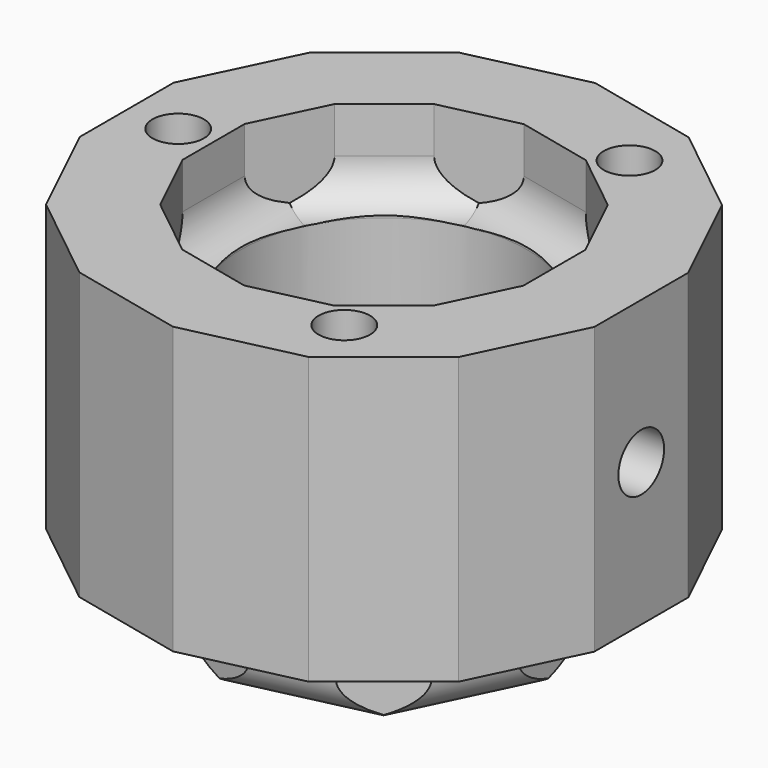
from build123d import *

# Parameters (mm, degrees)
F0_R         = 12.5
F1_DEPTH     = 12.5
F2_R         = 2.25
F3_DEPTH     = 25
F4_R         = 12.5
F5_DEPTH     = 7.5
F6_R         = 12.5
F7_DEPTH     = 7.5
F8_T4_DEPTH  = 24.3016555368
F8_S5_R      = 12.5
F8_T6_DEPTH  = 15
F8_T11_DEPTH = 24.3016555368
F8_S12_R     = 12.5
F8_T13_DEPTH = 14
F8_T17_DEPTH = 24.3016555368
F8_S18_R     = 12.5
F8_T19_DEPTH = 15
F8_T24_DEPTH = 24.3016555368
F8_S25_R     = 12.5
F8_T26_DEPTH = 15
F8_T30_DEPTH = 24.3016555368
F8_S31_R     = 12.5
F8_T32_DEPTH = 15
F8_T37_DEPTH = 24.3016555368
F8_S38_R     = 12.5
F8_T39_DEPTH = 15
F8_T44_DEPTH = 24.3016555368
F8_S45_R     = 12.5
F8_T46_DEPTH = 15
F9_T1_DEPTH  = 24.050587715
F9_T3_DEPTH  = 24.050587715
F9_T5_DEPTH  = 24.050587715
F9_T7_DEPTH  = 24.050587715
F9_T9_DEPTH  = 24.050587715
F9_T11_DEPTH = 24.050587715
F9_T13_DEPTH = 24.050587715
F10_R        = 2.5
F11_DEPTH    = 12


# Not quite as in the source:
# - a fillet or chamfer that OpenCascade refuses, or shapes differently, is made with other operations: its cross-section is extruded or revolved along the edge and cut away or added


with BuildPart() as f1:
    # F0 (on Top) → F1 (new body, symmetric)
    with BuildSketch(Plane.XY):
        Polygon((22.5, -5.1354781738), (22.5, 5.1354781738), (18.0435990556, 14.3892900865), (10.013442028, 20.7931266245), (0, 23.0786294236), (-10.013442028, 20.7931266245), (-18.0435990556, 14.3892900865), (-22.5, 5.1354781738), (-22.5, -5.1354781738), (-18.0435990556, -14.3892900865), (-10.013442028, -20.7931266245), (0, -23.0786294236), (10.013442028, -20.7931266245), (18.0435990556, -14.3892900865), align=None)
        Circle(F0_R, mode=Mode.SUBTRACT)
    extrude(amount=F1_DEPTH, both=True)

    # F2 (on face) → F3 (cut)
    with BuildSketch(Plane.XY.offset(12.5)):
        with Locations((9, 15.5884572681)):
            Circle(F2_R)
        with Locations((-18, 0)):
            Circle(F2_R)
        with Locations((9, -15.5884572681)):
            Circle(F2_R)
    extrude(amount=-F3_DEPTH, mode=Mode.SUBTRACT)

    # F4 (on face) → F5 (cut)
    with BuildSketch(Plane.XY.offset(12.5)):
        Polygon((14.9, -3.4008277684), (14.9, 3.4008277684), (11.9488722635, 9.5289076573), (6.6311238319, 13.7696705203), (0, 15.2831812628), (-6.6311238319, 13.7696705203), (-11.9488722635, 9.5289076573), (-14.9, 3.4008277684), (-14.9, -3.4008277684), (-11.9488722635, -9.5289076573), (-6.6311238319, -13.7696705203), (0, -15.2831812628), (6.6311238319, -13.7696705203), (11.9488722635, -9.5289076573), align=None)
        Circle(F4_R, mode=Mode.SUBTRACT)
    extrude(amount=-F5_DEPTH, mode=Mode.SUBTRACT)

    # F6 (on face) → F7 (join)
    with BuildSketch(Plane(origin=(0, 0, -12.5), x_dir=(1, 0, 0), z_dir=(0, 0, -1))):
        Polygon((14.35, -3.2752938575), (14.35, 3.2752938575), (11.5078065088, 9.1771694552), (6.3863508045, 13.2613940917), (0, 14.719036988), (-6.3863508045, 13.2613940917), (-11.5078065088, 9.1771694552), (-14.35, 3.2752938575), (-14.35, -3.2752938575), (-11.5078065088, -9.1771694552), (-6.3863508045, -13.2613940917), (0, -14.719036988), (6.3863508045, -13.2613940917), (11.5078065088, -9.1771694552), align=None)
        Circle(F6_R, mode=Mode.SUBTRACT)
    extrude(amount=F7_DEPTH)

    # F8: fillet of radius 3.5 on 7 edges, made by hand


with BuildPart() as f8_tool2:
    # F8_s3 → F8_t4 (new body)
    with BuildSketch(Plane(origin=(9.4998996874, 7.5759171977, 0), x_dir=(0, 0, 1), z_dir=(-0.7818314825, -0.6234898019, 0))):
        with BuildLine():
            ThreePointArc((5, 11.4), (6.0251262658, 13.8748737342), (8.5, 14.9))
            Line((8.5, 14.9), (5, 14.9))
            Line((5, 14.9), (5, 11.4))
        make_face()
    extrude(amount=F8_T4_DEPTH)

    # F8_s5 → F8_t6 (cut, symmetric)
    with BuildSketch(Plane.XY.offset(6.8)):
        Circle(F8_S5_R)
    extrude(amount=F8_T6_DEPTH, both=True, mode=Mode.SUBTRACT)

    split(bisect_by=Plane(origin=(-13.4244361317, 6.4648677129, 0), x_dir=(0, 0, 1), z_dir=(0.9009688679, -0.4338837391, 0)), keep=Keep.TOP)


with BuildPart() as f1_1:
    add(f1.part)

    # F8_t1: union F8_tool2
    add(f8_tool2.part)


with BuildPart() as f8_tool9:
    # F8_s10 → F8_t11 (new body)
    with BuildSketch(Plane.XZ.offset(-12.1508277684)):
        with BuildLine():
            ThreePointArc((-11.4, 5), (-13.8748737342, 6.0251262658), (-14.9, 8.5))
            Line((-14.9, 8.5), (-14.9, 5))
            Line((-14.9, 5), (-11.4, 5))
        make_face()
    extrude(amount=F8_T11_DEPTH)

    # F8_s12 → F8_t13 (cut, symmetric)
    with BuildSketch(Plane.XY.offset(6.8)):
        Circle(F8_S12_R)
    extrude(amount=F8_T13_DEPTH, both=True, mode=Mode.SUBTRACT)


with BuildPart() as f1_2:
    add(f1_1.part)

    # F8_t8: union F8_tool9
    add(f8_tool9.part)


with BuildPart() as f8_tool15:
    # F8_s16 → F8_t17 (new body)
    with BuildSketch(Plane(origin=(-9.4998996874, 7.5759171977, 0), x_dir=(0, 0, 1), z_dir=(0.7818314825, -0.6234898019, 0))):
        with BuildLine():
            ThreePointArc((5, 11.4), (6.0251262658, 13.8748737342), (8.5, 14.9))
            Line((8.5, 14.9), (5, 14.9))
            Line((5, 14.9), (5, 11.4))
        make_face()
    extrude(amount=F8_T17_DEPTH)

    # F8_s18 → F8_t19 (cut, symmetric)
    with BuildSketch(Plane.XY.offset(6.8)):
        Circle(F8_S18_R)
    extrude(amount=F8_T19_DEPTH, both=True, mode=Mode.SUBTRACT)

    split(bisect_by=Plane.YZ.offset(-14.9), keep=Keep.TOP)


with BuildPart() as f1_3:
    add(f1_2.part)

    # F8_t14: union F8_tool15
    add(f8_tool15.part)


with BuildPart() as f8_tool22:
    # F8_s23 → F8_t24 (new body)
    with BuildSketch(Plane(origin=(-11.8461811475, -2.7038135434, 0), x_dir=(0, 0, 1), z_dir=(0.9749279122, 0.222520934, 0))):
        with BuildLine():
            ThreePointArc((8.5, 14.9), (6.0251262658, 13.8748737342), (5, 11.4))
            Line((5, 11.4), (5, 14.9))
            Line((5, 14.9), (8.5, 14.9))
        make_face()
    extrude(amount=F8_T24_DEPTH)

    # F8_s25 → F8_t26 (cut, symmetric)
    with BuildSketch(Plane.XY.offset(6.8)):
        Circle(F8_S25_R)
    extrude(amount=F8_T26_DEPTH, both=True, mode=Mode.SUBTRACT)


with BuildPart() as f1_4:
    add(f1_3.part)

    # F8_t21: union F8_tool22
    add(f8_tool22.part)


with BuildPart() as f8_tool28:
    # F8_s29 → F8_t30 (new body)
    with BuildSketch(Plane(origin=(-5.2720465855, -10.9475175386, 0), x_dir=(0, 0, 1), z_dir=(0.4338837391, 0.9009688679, 0))):
        with BuildLine():
            ThreePointArc((5, 11.4), (6.0251262658, 13.8748737342), (8.5, 14.9))
            Line((8.5, 14.9), (5, 14.9))
            Line((5, 14.9), (5, 11.4))
        make_face()
    extrude(amount=F8_T30_DEPTH)

    # F8_s31 → F8_t32 (cut, symmetric)
    with BuildSketch(Plane.XY.offset(6.8)):
        Circle(F8_S31_R)
    extrude(amount=F8_T32_DEPTH, both=True, mode=Mode.SUBTRACT)

    split(bisect_by=Plane(origin=(9.2899980477, -11.6492890888, 0), x_dir=(0, 0, 1), z_dir=(-0.6234898019, 0.7818314825, 0)), keep=Keep.TOP)


with BuildPart() as f1_5:
    add(f1_4.part)

    # F8_t27: union F8_tool28
    add(f8_tool28.part)


with BuildPart() as f8_tool35:
    # F8_s36 → F8_t37 (new body)
    with BuildSketch(Plane(origin=(5.2720465855, -10.9475175386, 0), x_dir=(0, 0, 1), z_dir=(-0.4338837391, 0.9009688679, 0))):
        with BuildLine():
            ThreePointArc((5, 11.4), (6.0251262658, 13.8748737342), (8.5, 14.9))
            Line((8.5, 14.9), (5, 14.9))
            Line((5, 14.9), (5, 11.4))
        make_face()
    extrude(amount=F8_T37_DEPTH)

    # F8_s38 → F8_t39 (cut, symmetric)
    with BuildSketch(Plane.XY.offset(6.8)):
        Circle(F8_S38_R)
    extrude(amount=F8_T39_DEPTH, both=True, mode=Mode.SUBTRACT)

    split(bisect_by=Plane(origin=(9.2899980477, 11.6492890888, 0), x_dir=(0, 0, 1), z_dir=(-0.6234898019, -0.7818314825, 0)), keep=Keep.TOP)


with BuildPart() as f1_6:
    add(f1_5.part)

    # F8_t34: union F8_tool35
    add(f8_tool35.part)


with BuildPart() as f8_tool42:
    # F8_s43 → F8_t44 (new body)
    with BuildSketch(Plane(origin=(11.8461811475, -2.7038135434, 0), x_dir=(0, 0, 1), z_dir=(-0.9749279122, 0.222520934, 0))):
        with BuildLine():
            ThreePointArc((5, 11.4), (6.0251262658, 13.8748737342), (8.5, 14.9))
            Line((8.5, 14.9), (5, 14.9))
            Line((5, 14.9), (5, 11.4))
        make_face()
    extrude(amount=F8_T44_DEPTH)

    # F8_s45 → F8_t46 (cut, symmetric)
    with BuildSketch(Plane.XY.offset(6.8)):
        Circle(F8_S45_R)
    extrude(amount=F8_T46_DEPTH, both=True, mode=Mode.SUBTRACT)


with BuildPart() as f1_7:
    add(f1_6.part)

    # F8_t41: union F8_tool42
    add(f8_tool42.part)

    # F9: fillet of radius 3.5 on 7 edges, made by hand

    # F9_s2 → F9_t1 (cut)
    with BuildSketch(Plane(origin=(-5.2175794629, 10.834415393, 0), x_dir=(0, 0, 1), z_dir=(0.4338837391, -0.9009688679, 0))):
        with BuildLine():
            ThreePointArc((-16.5, -14.35), (-18.9748737342, -13.3248737342), (-20, -10.85))
            Line((-20, -10.85), (-20, -14.35))
            Line((-20, -14.35), (-16.5, -14.35))
        make_face()
    extrude(amount=F9_T1_DEPTH, mode=Mode.SUBTRACT)

    # F9_s4 → F9_t3 (cut)
    with BuildSketch(Plane(origin=(-11.7237946339, 2.6758796203, 0), x_dir=(0, 0, 1), z_dir=(0.9749279122, -0.222520934, 0))):
        with BuildLine():
            ThreePointArc((-16.5, -14.35), (-18.9748737342, -13.3248737342), (-20, -10.85))
            Line((-20, -10.85), (-20, -14.35))
            Line((-20, -14.35), (-16.5, -14.35))
        make_face()
    extrude(amount=F9_T3_DEPTH, mode=Mode.SUBTRACT)

    # F9_s6 → F9_t5 (cut)
    with BuildSketch(Plane(origin=(-9.4017533237, -7.4976480845, 0), x_dir=(0, 0, 1), z_dir=(0.7818314825, 0.6234898019, 0))):
        with BuildLine():
            ThreePointArc((-16.5, -14.35), (-18.9748737342, -13.3248737342), (-20, -10.85))
            Line((-20, -10.85), (-20, -14.35))
            Line((-20, -14.35), (-16.5, -14.35))
        make_face()
    extrude(amount=F9_T5_DEPTH, mode=Mode.SUBTRACT)

    # F9_s8 → F9_t7 (cut)
    with BuildSketch(Plane.XZ.offset(-12.0252938575)):
        with BuildLine():
            ThreePointArc((-14.35, -16.5), (-13.3248737342, -18.9748737342), (-10.85, -20))
            Line((-10.85, -20), (-14.35, -20))
            Line((-14.35, -20), (-14.35, -16.5))
        make_face()
    extrude(amount=F9_T7_DEPTH, mode=Mode.SUBTRACT)

    # F9_s10 → F9_t9 (cut)
    with BuildSketch(Plane(origin=(9.4017533237, -7.4976480845, 0), x_dir=(0, 0, 1), z_dir=(-0.7818314825, 0.6234898019, 0))):
        with BuildLine():
            ThreePointArc((-16.5, -14.35), (-18.9748737342, -13.3248737342), (-20, -10.85))
            Line((-20, -10.85), (-20, -14.35))
            Line((-20, -14.35), (-16.5, -14.35))
        make_face()
    extrude(amount=F9_T9_DEPTH, mode=Mode.SUBTRACT)

    # F9_s12 → F9_t11 (cut)
    with BuildSketch(Plane(origin=(11.7237946339, 2.6758796203, 0), x_dir=(0, 0, 1), z_dir=(-0.9749279122, -0.222520934, 0))):
        with BuildLine():
            ThreePointArc((-16.5, -14.35), (-18.9748737342, -13.3248737342), (-20, -10.85))
            Line((-20, -10.85), (-20, -14.35))
            Line((-20, -14.35), (-16.5, -14.35))
        make_face()
    extrude(amount=F9_T11_DEPTH, mode=Mode.SUBTRACT)

    # F9_s14 → F9_t13 (cut)
    with BuildSketch(Plane(origin=(5.2175794629, 10.834415393, 0), x_dir=(0, 0, 1), z_dir=(-0.4338837391, -0.9009688679, 0))):
        with BuildLine():
            ThreePointArc((-16.5, -14.35), (-18.9748737342, -13.3248737342), (-20, -10.85))
            Line((-20, -10.85), (-20, -14.35))
            Line((-20, -14.35), (-16.5, -14.35))
        make_face()
    extrude(amount=F9_T13_DEPTH, mode=Mode.SUBTRACT)

    # F10 (on face) → F11 (cut)
    with BuildSketch(Plane.YZ.offset(22.5)):
        Circle(F10_R)
    extrude(amount=-F11_DEPTH, mode=Mode.SUBTRACT)


solid = f1_7.part
